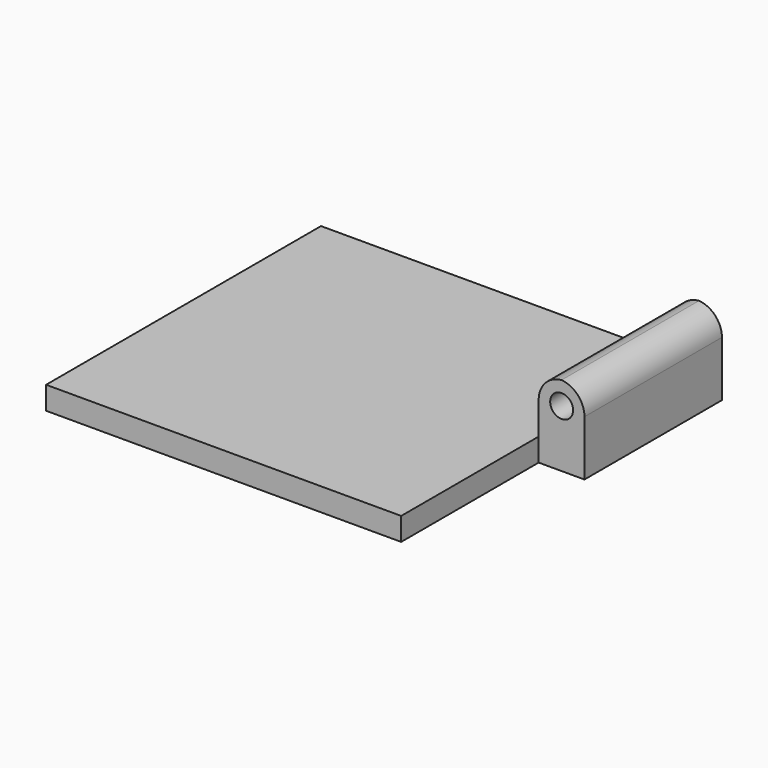
from build123d import *

# Parameters (mm, degrees)
F0_W        = 35
F0_H        = 30
F1_DEPTH    = 2
F2_W        = 4
F2_H        = 15
F3_DEPTH    = 5
F4_R        = 1
F5_DEPTH    = 25
F6_T1_DEPTH = 25.8639610307
F7_W        = 4
F7_H        = 15
F8_DEPTH    = 25


# Not quite as in the source:
# - a fillet or chamfer that OpenCascade refuses, or shapes differently, is made with other operations: its cross-section is extruded or revolved along the edge and cut away or added


with BuildPart() as f1:
    # F0 (on Top) → F1 (new body)
    with BuildSketch(Plane.XY):
        with Locations((-17.5, 0)):
            Rectangle(F0_W, F0_H)
    extrude(amount=F1_DEPTH)

    # F2 (on face) → F3 (join)
    with BuildSketch(Plane.XY.offset(2)):
        with Locations((-2, 7.5)):
            Rectangle(F2_W, F2_H)
    extrude(amount=F3_DEPTH)

    # F4 (on face) → F5 (cut)
    with BuildSketch(Plane.XZ):
        with Locations((-1.9937221408, 4.9999934314)):
            Circle(F4_R)
    extrude(amount=-F5_DEPTH, mode=Mode.SUBTRACT)

    # F6: fillet of radius 2.1727922061 on 2 edges, made by hand

    # F6_s2 → F6_t1 (cut)
    with BuildSketch(Plane.XZ.offset(-20.4319805153)):
        with BuildLine():
            ThreePointArc((-1.8272077939, 7), (-3.3636038969, 6.3636038969), (-4, 4.8272077939))
            Line((-4, 4.8272077939), (-4, 7))
            Line((-4, 7), (-1.8272077939, 7))
        make_face()
        with BuildLine():
            ThreePointArc((0, 4.8272077939), (-0.6363961031, 6.3636038969), (-2.1727922061, 7))
            Line((-2.1727922061, 7), (0, 7))
            Line((0, 7), (0, 4.8272077939))
        make_face()
    extrude(amount=F6_T1_DEPTH, mode=Mode.SUBTRACT)

    # F7 (on face) → F8 (cut)
    with BuildSketch(Plane.XY.offset(2)):
        with Locations((-2, -7.5)):
            Rectangle(F7_W, F7_H)
    extrude(amount=-F8_DEPTH, mode=Mode.SUBTRACT)


solid = f1.part
